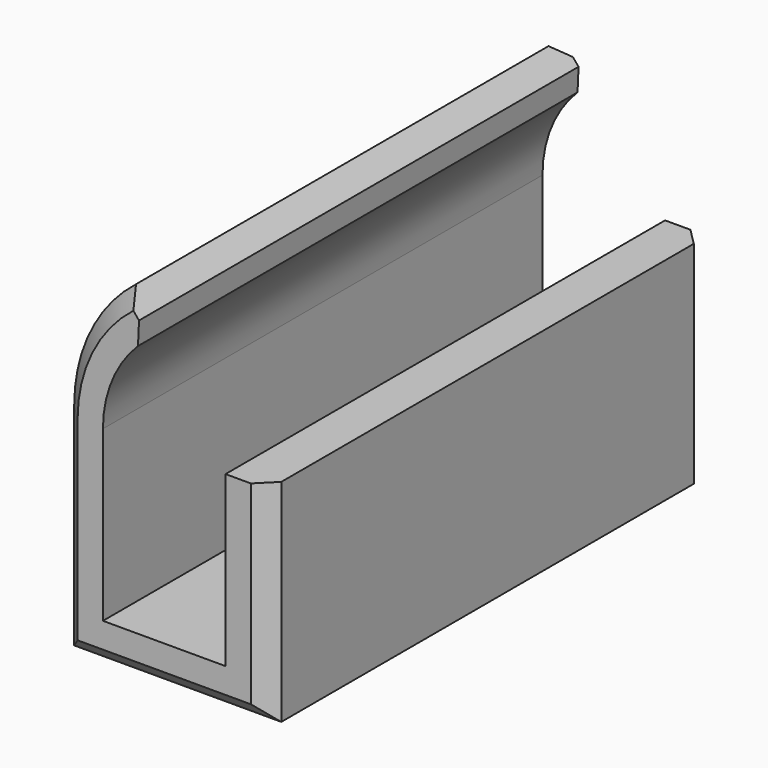
from build123d import *

# Parameters (mm, degrees)
F1_DEPTH     = 13
F2_T1_DEPTH  = 6.0286731952
F2_T3_DEPTH  = 15.0178646599
F2_T5_DEPTH  = 6.9573463904
F2_T7_DEPTH  = 7.0573463904
F2_T10_ANGLE = 67.461453667
F2_T12_ANGLE = 67.461453667


# Not quite as in the source:
# - a fillet or chamfer that OpenCascade refuses, or shapes differently, is made with other operations: its cross-section is extruded or revolved along the edge and cut away or added


with BuildPart() as f1:
    # F0 (on Front) → F1 (new body)
    with BuildSketch(Plane.XZ):
        with BuildLine():
            Line((0, 5), (0, 0))
            Line((0, 0), (4.9, 0))
            Line((4.9, 0), (4.9, 5))
            Line((4.9, 5), (3.9, 5))
            Line((3.9, 5), (3.9, 1))
            Line((3.9, 1), (1, 1))
            Line((1, 1), (1, 5))
            ThreePointArc((1, 5), (1.2914644914, 6.2462400161), (2.1053955316, 7.2339555569))
            Line((2.1053955316, 7.2339555569), (1.4626079219, 8))
            ThreePointArc((1.4626079219, 8), (0.3851271545, 6.6687736465), (0, 5))
        make_face()
    extrude(amount=F1_DEPTH)

    # F2: chamfer of 0.4 on 9 edges, made by hand

    # F2_s2 → F2_t1 (cut)
    with BuildSketch(Plane.XY.offset(-1.0286731952)):
        Polygon((0, -12.6), (0.4, -13), (0, -13), align=None)
        Polygon((0, -0.4), (0.4, 0), (0, 0), align=None)
    extrude(amount=F2_T1_DEPTH, mode=Mode.SUBTRACT)

    # F2_s4 → F2_t3 (cut)
    with BuildSketch(Plane.XZ.offset(-1.00893233)):
        with BuildLine():
            Line((1.8291984844, 6.9931446867), (1.8536490905, 7.5339752825))
            Line((1.8536490905, 7.5339752825), (2.1053955316, 7.2339555569))
            ThreePointArc((2.1053955316, 7.2339555569), (1.9591897538, 7.1144071406), (1.8291984844, 6.9931446867))
        make_face()
    extrude(amount=F2_T3_DEPTH, mode=Mode.SUBTRACT)

    # F2_s6 → F2_t5 (cut)
    with BuildSketch(Plane.YZ.offset(-1.0286731952)):
        Polygon((-0.4, 0), (0, 0.4), (0, 0), align=None)
        Polygon((-12.6, 0), (-13, 0.4), (-13, 0), align=None)
    extrude(amount=F2_T5_DEPTH, mode=Mode.SUBTRACT)

    # F2_s8 → F2_t7 (cut)
    with BuildSketch(Plane.XY.offset(-1.0286731952)):
        Polygon((4.9, -0.4), (4.5, 0), (4.9, 0), align=None)
        Polygon((4.9, -12.6), (4.5, -13), (4.9, -13), align=None)
    extrude(amount=F2_T7_DEPTH, mode=Mode.SUBTRACT)

    # F2_s9 → F2_t10 (revolve, cut)
    with BuildSketch(Plane(origin=(5.0186624957, 0, 2.0827548228), x_dir=(0, 1, 0), z_dir=(0.9236218692, 0, 0.3833048953))):
        Polygon((-0.4, 6.9664843046), (0, 6.5664843046), (0, 6.9664843046), align=None)
    revolve(axis=Axis((3.808, 0, 5), (0, -1, 0)), revolution_arc=F2_T10_ANGLE, mode=Mode.SUBTRACT)

    # F2_s11 → F2_t12 (revolve, cut)
    with BuildSketch(Plane(origin=(5.0186624957, 0, 2.0827548228), x_dir=(0, 1, 0), z_dir=(0.9236218692, 0, 0.3833048953))):
        Polygon((-12.6, 6.9664843046), (-13, 6.5664843046), (-13, 6.9664843046), align=None)
    revolve(axis=Axis((3.808, -13, 5), (0, -1, 0)), revolution_arc=F2_T12_ANGLE, mode=Mode.SUBTRACT)


solid = f1.part
